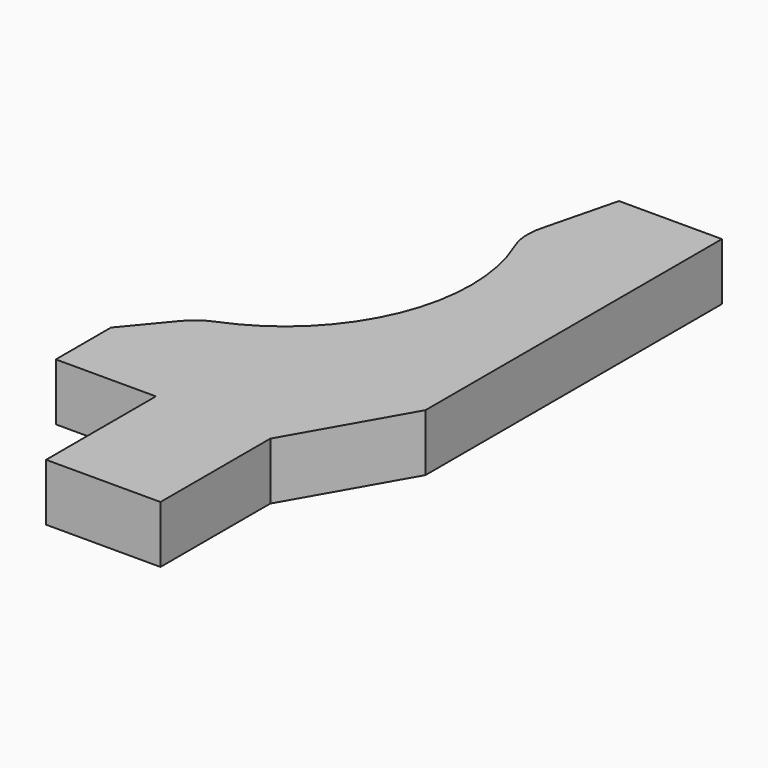
from build123d import *

# Parameters (mm, degrees)
F1_DEPTH = 5


# Not quite as in the source:
# - ends of sketch curves that miss each other by under 0.0002 mm in the source are joined


with BuildPart() as f1:
    # F0 (on Top) → F1 (new body)
    with BuildSketch(Plane.XY):
        with BuildLine():
            ThreePointArc((1.8058852177, 17.4790926703), (1.8279530148, 4.8720604744), (-7.149820085, -3.9787777878))
            ThreePointArc((-7.149820085, -3.9787777878), (-8.2306223723, -4.5782907715), (-9.1313488192, -5.4246011501))
            Line((-9.1313488192, -5.4246011501), (-12.197101, -9.119353))
            Line((-12.197101, -9.119353), (-12.197101, -15.150279))
            Line((-12.197101, -15.150279), (-3.447101, -15.150279))
            Line((-3.447101, -15.150279), (-3.447101, -27.150279))
            Line((-3.447101, -27.150279), (6.552899, -27.150279))
            Line((6.552899, -27.150279), (6.552899, -15.150279))
            Line((6.552899, -15.150279), (12.197102, -5.240307))
            Line((12.197102, -5.240307), (12.197102, 27.150279))
            Line((12.197102, 27.150279), (3.197102, 27.150279))
            Line((3.197102, 27.150279), (1.562377, 20.643277))
            ThreePointArc((1.562377, 20.643277), (1.4264287194, 19.0413526341), (1.8058852177, 17.4790926703))
        make_face()
    extrude(amount=F1_DEPTH)


solid = f1.part
